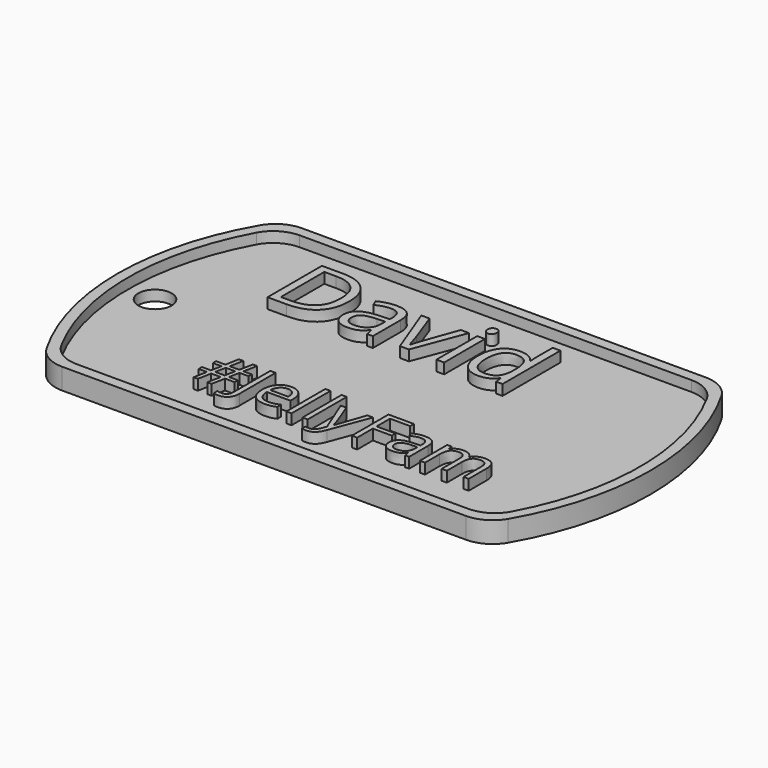
from build123d import *

# Parameters (mm, degrees)
F1_DEPTH       = 1
F3_DEPTH       = 1
F4_R           = 1.5875
F5_DEPTH       = 1
F6_TEXT_SIZE   = 9.0744469263
F6_TEXT_SIZE_2 = 6.1083009415
F7_DEPTH       = 1


# Not quite as in the source:
# - a feature of the source that left no trace in its solid (it failed there, or was rolled back) is left out
# - Text() gives the source's letters only with a copy of the font that has no kerning and outlines rounded to 1/6400 em; it was checked with that copy


with BuildPart() as f1:
    # F0 (on Top) → F1 (new body)
    with BuildSketch(Plane.XY):
        with BuildLine():
            ThreePointArc((-19.2474145991, 14.2875), (-20.8349145991, 13.862130657), (-21.9970452561, 12.7))
            ThreePointArc((-21.9970452561, 12.7), (-25.4, 0), (-21.9970452561, -12.7))
            ThreePointArc((-21.9970452561, -12.7), (-20.8349145991, -13.862130657), (-19.2474145991, -14.2875))
            Line((-19.2474145991, -14.2875), (19.2474145991, -14.2875))
            ThreePointArc((19.2474145991, -14.2875), (20.8349145991, -13.862130657), (21.9970452561, -12.7))
            ThreePointArc((21.9970452561, -12.7), (25.4, 0), (21.9970452561, 12.7))
            ThreePointArc((21.9970452561, 12.7), (20.8349145991, 13.862130657), (19.2474145991, 14.2875))
            Line((19.2474145991, 14.2875), (-19.2474145991, 14.2875))
        make_face()
    extrude(amount=F1_DEPTH)

    # F2 (on face) → F3 (join)
    with BuildSketch(Plane.XY.offset(1)):
        with BuildLine():
            Line((19.2474145991, 14.2875), (-19.2474145991, 14.2875))
            ThreePointArc((-19.2474145991, 14.2875), (-20.8349145991, 13.862130657), (-21.9970452561, 12.7))
            ThreePointArc((-21.9970452561, 12.7), (-25.4, 0), (-21.9970452561, -12.7))
            ThreePointArc((-21.9970452561, -12.7), (-20.8349145991, -13.862130657), (-19.2474145991, -14.2875))
            Line((-19.2474145991, -14.2875), (19.2474145991, -14.2875))
            ThreePointArc((19.2474145991, -14.2875), (20.8349145991, -13.862130657), (21.9970452561, -12.7))
            ThreePointArc((21.9970452561, -12.7), (25.4, 0), (21.9970452561, 12.7))
            ThreePointArc((21.9970452561, 12.7), (20.8349145991, 13.862130657), (19.2474145991, 14.2875))
        make_face()
        with BuildLine():
            ThreePointArc((-21.4526124879, 11.6252061249), (-20.2856017842, 12.8404540819), (-18.6611352482, 13.2875))
            Line((-18.6611352482, 13.2875), (18.6611352482, 13.2875))
            ThreePointArc((18.6611352482, 13.2875), (20.2856017842, 12.8404540819), (21.4526124879, 11.6252061249))
            ThreePointArc((21.4526124879, 11.6252061249), (24.4, 0), (21.4526124879, -11.6252061249))
            ThreePointArc((21.4526124879, -11.6252061249), (20.2856017842, -12.8404540819), (18.6611352482, -13.2875))
            Line((18.6611352482, -13.2875), (-18.6611352482, -13.2875))
            ThreePointArc((-18.6611352482, -13.2875), (-20.2856017842, -12.8404540819), (-21.4526124879, -11.6252061249))
            ThreePointArc((-21.4526124879, -11.6252061249), (-24.4, 0), (-21.4526124879, 11.6252061249))
        make_face(mode=Mode.SUBTRACT)
    extrude(amount=F3_DEPTH)

    # F4 (on face) → F5 (cut)
    with BuildSketch(Plane.XY.offset(1)):
        with Locations((-21.821282804, 0)):
            Circle(F4_R)
    extrude(amount=-F5_DEPTH, mode=Mode.SUBTRACT)

    # F6 (on face) → F7 (join)
    with BuildSketch(Plane.XY.offset(1)):
        with Locations((-15.1945482939, 4.0053925477)):
            Text('David', F6_TEXT_SIZE, font='Open Sans', text_align=(TextAlign.LEFT, TextAlign.BOTTOM))
        with Locations((-11.2400883809, -9.4942576252)):
            Text('#JellyFam', F6_TEXT_SIZE_2, font='Open Sans', text_align=(TextAlign.LEFT, TextAlign.BOTTOM))
    extrude(amount=F7_DEPTH)


solid = f1.part
